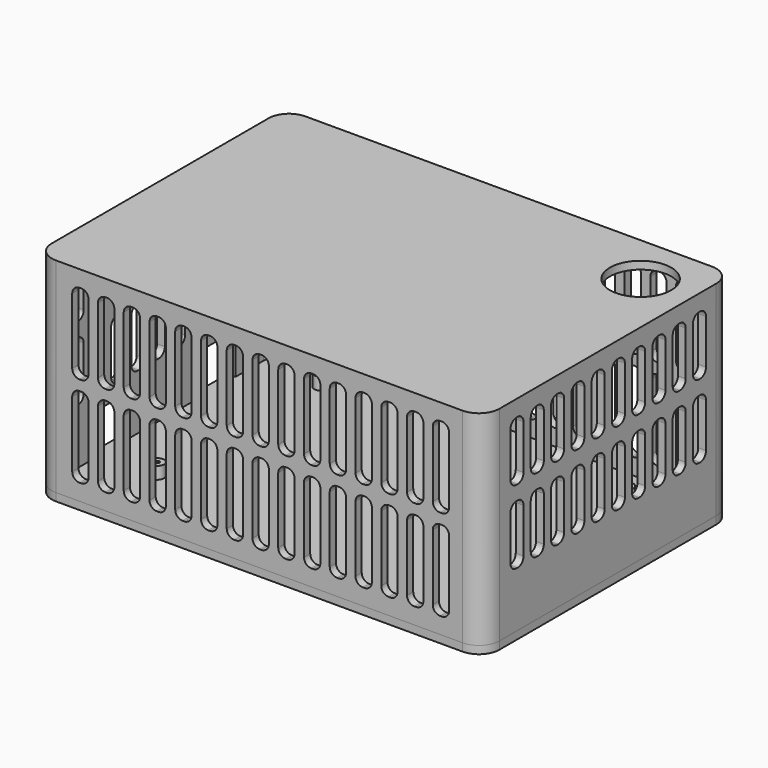
from build123d import *

# Parameters (mm, degrees)
F2_W         = 109.505
F2_H         = 76.3
F3_DEPTH     = 50
F4_T         = -1.905
F5_DEPTH     = 1.905
F0_W         = 9.525
F0_H         = 11.43
F0_W_2       = 6.35
F6_DEPTH     = 10
F0_W_3       = 11.43
F0_H_2       = 8.4328
F0_W_4       = 1.905
F7_DEPTH     = 10
F0_R         = 1.5875
F0_R_2       = 1.59
F8_DEPTH     = 3
F10_D        = 3.3
F12_D        = 1
F12_DEPTH    = 3
F12_TIP      = 0.3004303095
F13_DEPTH    = 5
F14_D        = 1
F14_DEPTH    = 3
F14_TIP      = 0.3004303095
F15_T1_DEPTH = 5
F16_R        = 5
F16_2_R      = 5
F18_DEPTH    = 76.301
F20_DEPTH    = 109.506
F21_R        = 7.5
F22_DEPTH    = 51.906


# Not quite as in the source:
# - a fillet or chamfer that OpenCascade refuses, or shapes differently, is made with other operations: its cross-section is extruded or revolved along the edge and cut away or added


with BuildPart() as f3:
    # F2 (on Top) → F3 (new body)
    with BuildSketch(Plane.XY):
        with Locations((16.3090971484, -6.4307405627)):
            Rectangle(F2_W, F2_H)
    extrude(amount=F3_DEPTH)

    # F4
    f4_openings = [f3.faces().sort_by_distance(p)[0] for p in [
        (16.309097, -6.430741, 0),
    ]]
    offset(amount=F4_T, openings=f4_openings)

    # F0 (on Top) → F6 (cut)
    with BuildSketch(Plane.XY):
        with Locations((-31.7759028516, 8.4792594373)):
            Rectangle(F0_W, F0_H)
        with Locations((-39.7134028516, 8.4792594373)):
            Rectangle(F0_W_2, F0_H)
    extrude(amount=F6_DEPTH, mode=Mode.SUBTRACT)

    # F0 (on Top) → F7 (cut)
    with BuildSketch(Plane.XY):
        with Locations((-30.8234028516, -22.2293405627)):
            Rectangle(F0_W_3, F0_H_2)
        with Locations((-37.4909028516, -22.2293405627)):
            Rectangle(F0_W_4, F0_H_2)
    extrude(amount=F7_DEPTH, mode=Mode.SUBTRACT)

    # F9 (on face) → F13 (join)
    with BuildSketch(Plane.XY):
        with BuildLine():
            ThreePointArc((69.5615971484, 27.7192594373), (67.0615971484, 30.2192594373), (64.5615971484, 27.7192594373))
            Line((64.5615971484, 27.7192594373), (67.0615971484, 27.7192594373))
            Line((67.0615971484, 27.7192594373), (67.0615971484, 25.2192594373))
            ThreePointArc((67.0615971484, 25.2192594373), (68.8293641014, 25.9514924844), (69.5615971484, 27.7192594373))
        make_face()
        with BuildLine():
            Line((67.0615971484, 27.7192594373), (64.5615971484, 27.7192594373))
            ThreePointArc((64.5615971484, 27.7192594373), (65.2938301955, 25.9514924844), (67.0615971484, 25.2192594373))
            Line((67.0615971484, 25.2192594373), (67.0615971484, 27.7192594373))
        make_face()
        with BuildLine():
            Line((67.0615971484, -40.5807405627), (67.0615971484, -38.0807405627))
            ThreePointArc((67.0615971484, -38.0807405627), (65.2938301955, -38.8129736097), (64.5615971484, -40.5807405627))
            Line((64.5615971484, -40.5807405627), (67.0615971484, -40.5807405627))
        make_face()
        with BuildLine():
            ThreePointArc((69.5615971484, -40.5807405627), (68.8293641014, -38.8129736097), (67.0615971484, -38.0807405627))
            Line((67.0615971484, -38.0807405627), (67.0615971484, -40.5807405627))
            Line((67.0615971484, -40.5807405627), (64.5615971484, -40.5807405627))
            ThreePointArc((64.5615971484, -40.5807405627), (67.0615971484, -43.0807405627), (69.5615971484, -40.5807405627))
        make_face()
        with BuildLine():
            Line((-34.4434028516, 27.7192594373), (-31.9434028516, 27.7192594373))
            ThreePointArc((-31.9434028516, 27.7192594373), (-36.2111698045, 29.4870263903), (-34.4434028516, 25.2192594373))
            Line((-34.4434028516, 25.2192594373), (-34.4434028516, 27.7192594373))
        make_face()
        with BuildLine():
            ThreePointArc((-34.4434028516, 25.2192594373), (-32.6756358986, 25.9514924844), (-31.9434028516, 27.7192594373))
            Line((-31.9434028516, 27.7192594373), (-34.4434028516, 27.7192594373))
            Line((-34.4434028516, 27.7192594373), (-34.4434028516, 25.2192594373))
        make_face()
        with BuildLine():
            ThreePointArc((-31.9434028516, -40.5807405627), (-32.6756358986, -38.8129736097), (-34.4434028516, -38.0807405627))
            Line((-34.4434028516, -38.0807405627), (-34.4434028516, -40.5807405627))
            Line((-34.4434028516, -40.5807405627), (-31.9434028516, -40.5807405627))
        make_face()
        with BuildLine():
            Line((-34.4434028516, -40.5807405627), (-34.4434028516, -38.0807405627))
            ThreePointArc((-34.4434028516, -38.0807405627), (-36.2111698045, -42.3485075156), (-31.9434028516, -40.5807405627))
            Line((-31.9434028516, -40.5807405627), (-34.4434028516, -40.5807405627))
        make_face()
    extrude(amount=F13_DEPTH)

    # F14
    with Locations(Plane(origin=(0, 0, 0), x_dir=(1, 0, 0), z_dir=(0, 0, -1))):
        with Locations((-34.4434028516, 40.5807405627), (67.0615971484, 40.5807405627), (-34.4434028516, -27.7192594373), (67.0615971484, -27.7192594373)):
            Hole(F14_D / 2, depth=F14_DEPTH)
            with Locations((0, 0, -(F14_DEPTH + F14_TIP / 2))):  # 118° drill point
                Cone(0, F14_D / 2, F14_TIP, mode=Mode.SUBTRACT)

    # F15: fillet of radius 2.5 on 8 edges, made by hand

    # F15_s2 → F15_t1 (join)
    with BuildSketch(Plane.XY):
        with BuildLine():
            ThreePointArc((66.8590971484, -38.0889553091), (68.494564776, -37.2918307885), (69.1565971484, -35.5971700555))
            Line((69.1565971484, -35.5971700555), (69.1565971484, -39.2165649875))
            ThreePointArc((69.1565971484, -39.2165649875), (68.163080221, -38.3364734126), (66.8590971484, -38.0889553091))
        make_face()
        with BuildLine():
            ThreePointArc((62.0780266412, -42.6757405627), (63.7726873742, -42.0137081902), (64.5698118948, -40.3782405627))
            ThreePointArc((64.5698118948, -40.3782405627), (64.8173299984, -41.6822236353), (65.6974215732, -42.6757405627))
            Line((65.6974215732, -42.6757405627), (62.0780266412, -42.6757405627))
        make_face()
        with BuildLine():
            ThreePointArc((69.1565971484, 22.7356889301), (68.494564776, 24.4303496632), (66.8590971484, 25.2274741837))
            ThreePointArc((66.8590971484, 25.2274741837), (68.163080221, 25.4749922873), (69.1565971484, 26.3550838621))
            Line((69.1565971484, 26.3550838621), (69.1565971484, 22.7356889301))
        make_face()
        with BuildLine():
            ThreePointArc((64.5698118948, 27.5167594373), (63.7726873742, 29.1522270649), (62.0780266412, 29.8142594373))
            Line((62.0780266412, 29.8142594373), (65.6974215732, 29.8142594373))
            ThreePointArc((65.6974215732, 29.8142594373), (64.8173299984, 28.8207425099), (64.5698118948, 27.5167594373))
        make_face()
        with BuildLine():
            ThreePointArc((-36.5384028516, 22.7356889301), (-35.8763704792, 24.4303496632), (-34.2409028516, 25.2274741837))
            ThreePointArc((-34.2409028516, 25.2274741837), (-35.5448859242, 25.4749922873), (-36.5384028516, 26.3550838621))
            Line((-36.5384028516, 26.3550838621), (-36.5384028516, 22.7356889301))
        make_face()
        with BuildLine():
            ThreePointArc((-36.5384028516, -35.5971700555), (-35.8763704792, -37.2918307885), (-34.2409028516, -38.0889553091))
            ThreePointArc((-34.2409028516, -38.0889553091), (-35.5448859242, -38.3364734126), (-36.5384028516, -39.2165649875))
            Line((-36.5384028516, -39.2165649875), (-36.5384028516, -35.5971700555))
        make_face()
        with BuildLine():
            ThreePointArc((-31.951617598, -40.3782405627), (-31.1544930774, -42.0137081902), (-29.4598323444, -42.6757405627))
            Line((-29.4598323444, -42.6757405627), (-33.0792272764, -42.6757405627))
            ThreePointArc((-33.0792272764, -42.6757405627), (-32.1991357015, -41.6822236353), (-31.951617598, -40.3782405627))
        make_face()
        with BuildLine():
            ThreePointArc((-29.4598323444, 29.8142594373), (-31.1544930774, 29.1522270649), (-31.951617598, 27.5167594373))
            ThreePointArc((-31.951617598, 27.5167594373), (-32.1991357015, 28.8207425099), (-33.0792272764, 29.8142594373))
            Line((-33.0792272764, 29.8142594373), (-29.4598323444, 29.8142594373))
        make_face()
    extrude(amount=F15_T1_DEPTH)

    # F16
    f16_edges = [f3.edges().sort_by_distance(p)[0] for p in [
        (-38.443403, -44.580741, 25),
        (71.061597, -44.580741, 25),
        (-38.443403, 31.719259, 25),
        (71.061597, 31.719259, 25),
    ]]
    fillet(f16_edges, radius=F16_R)

    # F17 (on face) → F18 (cut, through all)
    with BuildSketch(Plane.XZ.offset(44.5807405627)):
        with BuildLine():
            Line((-27.2434028516, 46), (-27.6434028516, 46))
            ThreePointArc((-27.6434028516, 46), (-28.9161950577, 45.4727922061), (-29.4434028516, 44.2))
            Line((-29.4434028516, 44.2), (-29.4434028516, 28.05))
            ThreePointArc((-29.4434028516, 28.05), (-28.9161950577, 26.7772077939), (-27.6434028516, 26.25))
            Line((-27.6434028516, 26.25), (-27.2434028516, 26.25))
            ThreePointArc((-27.2434028516, 26.25), (-25.9706106454, 26.7772077939), (-25.4434028516, 28.05))
            Line((-25.4434028516, 28.05), (-25.4434028516, 44.2))
            ThreePointArc((-25.4434028516, 44.2), (-25.9706106454, 45.4727922061), (-27.2434028516, 46))
        make_face()
        with BuildLine():
            Line((-20.9434028516, 46), (-21.3434028516, 46))
            ThreePointArc((-21.3434028516, 46), (-22.6161950577, 45.4727922061), (-23.1434028516, 44.2))
            Line((-23.1434028516, 44.2), (-23.1434028516, 28.05))
            ThreePointArc((-23.1434028516, 28.05), (-22.6161950577, 26.7772077939), (-21.3434028516, 26.25))
            Line((-21.3434028516, 26.25), (-20.9434028516, 26.25))
            ThreePointArc((-20.9434028516, 26.25), (-19.6706106454, 26.7772077939), (-19.1434028516, 28.05))
            Line((-19.1434028516, 28.05), (-19.1434028516, 44.2))
            ThreePointArc((-19.1434028516, 44.2), (-19.6706106454, 45.4727922061), (-20.9434028516, 46))
        make_face()
        with BuildLine():
            Line((-14.6434028516, 46), (-15.0434028516, 46))
            ThreePointArc((-15.0434028516, 46), (-16.3161950577, 45.4727922061), (-16.8434028516, 44.2))
            Line((-16.8434028516, 44.2), (-16.8434028516, 28.05))
            ThreePointArc((-16.8434028516, 28.05), (-16.3161950577, 26.7772077939), (-15.0434028516, 26.25))
            Line((-15.0434028516, 26.25), (-14.6434028516, 26.25))
            ThreePointArc((-14.6434028516, 26.25), (-13.3706106454, 26.7772077939), (-12.8434028516, 28.05))
            Line((-12.8434028516, 28.05), (-12.8434028516, 44.2))
            ThreePointArc((-12.8434028516, 44.2), (-13.3706106454, 45.4727922061), (-14.6434028516, 46))
        make_face()
        with BuildLine():
            Line((-8.3434028516, 46), (-8.7434028516, 46))
            ThreePointArc((-8.7434028516, 46), (-10.0161950577, 45.4727922061), (-10.5434028516, 44.2))
            Line((-10.5434028516, 44.2), (-10.5434028516, 28.05))
            ThreePointArc((-10.5434028516, 28.05), (-10.0161950577, 26.7772077939), (-8.7434028516, 26.25))
            Line((-8.7434028516, 26.25), (-8.3434028516, 26.25))
            ThreePointArc((-8.3434028516, 26.25), (-7.0706106454, 26.7772077939), (-6.5434028516, 28.05))
            Line((-6.5434028516, 28.05), (-6.5434028516, 44.2))
            ThreePointArc((-6.5434028516, 44.2), (-7.0706106454, 45.4727922061), (-8.3434028516, 46))
        make_face()
        with BuildLine():
            Line((-2.0434028516, 46), (-2.4434028516, 46))
            ThreePointArc((-2.4434028516, 46), (-3.7161950577, 45.4727922061), (-4.2434028516, 44.2))
            Line((-4.2434028516, 44.2), (-4.2434028516, 28.05))
            ThreePointArc((-4.2434028516, 28.05), (-3.7161950577, 26.7772077939), (-2.4434028516, 26.25))
            Line((-2.4434028516, 26.25), (-2.0434028516, 26.25))
            ThreePointArc((-2.0434028516, 26.25), (-0.7706106454, 26.7772077939), (-0.2434028516, 28.05))
            Line((-0.2434028516, 28.05), (-0.2434028516, 44.2))
            ThreePointArc((-0.2434028516, 44.2), (-0.7706106454, 45.4727922061), (-2.0434028516, 46))
        make_face()
        with BuildLine():
            Line((4.2565971484, 46), (3.8565971484, 46))
            ThreePointArc((3.8565971484, 46), (2.5838049423, 45.4727922061), (2.0565971484, 44.2))
            Line((2.0565971484, 44.2), (2.0565971484, 28.05))
            ThreePointArc((2.0565971484, 28.05), (2.5838049423, 26.7772077939), (3.8565971484, 26.25))
            Line((3.8565971484, 26.25), (4.2565971484, 26.25))
            ThreePointArc((4.2565971484, 26.25), (5.5293893546, 26.7772077939), (6.0565971484, 28.05))
            Line((6.0565971484, 28.05), (6.0565971484, 44.2))
            ThreePointArc((6.0565971484, 44.2), (5.5293893546, 45.4727922061), (4.2565971484, 46))
        make_face()
        with BuildLine():
            Line((10.5565971484, 46), (10.1565971484, 46))
            ThreePointArc((10.1565971484, 46), (8.8838049423, 45.4727922061), (8.3565971484, 44.2))
            Line((8.3565971484, 44.2), (8.3565971484, 28.05))
            ThreePointArc((8.3565971484, 28.05), (8.8838049423, 26.7772077939), (10.1565971484, 26.25))
            Line((10.1565971484, 26.25), (10.5565971484, 26.25))
            ThreePointArc((10.5565971484, 26.25), (11.8293893546, 26.7772077939), (12.3565971484, 28.05))
            Line((12.3565971484, 28.05), (12.3565971484, 44.2))
            ThreePointArc((12.3565971484, 44.2), (11.8293893546, 45.4727922061), (10.5565971484, 46))
        make_face()
        with BuildLine():
            Line((16.8565971484, 46), (16.4565971484, 46))
            ThreePointArc((16.4565971484, 46), (15.1838049423, 45.4727922061), (14.6565971484, 44.2))
            Line((14.6565971484, 44.2), (14.6565971484, 28.05))
            ThreePointArc((14.6565971484, 28.05), (15.1838049423, 26.7772077939), (16.4565971484, 26.25))
            Line((16.4565971484, 26.25), (16.8565971484, 26.25))
            ThreePointArc((16.8565971484, 26.25), (18.1293893546, 26.7772077939), (18.6565971484, 28.05))
            Line((18.6565971484, 28.05), (18.6565971484, 44.2))
            ThreePointArc((18.6565971484, 44.2), (18.1293893546, 45.4727922061), (16.8565971484, 46))
        make_face()
        with BuildLine():
            Line((23.1565971484, 46), (22.7565971484, 46))
            ThreePointArc((22.7565971484, 46), (21.4838049423, 45.4727922061), (20.9565971484, 44.2))
            Line((20.9565971484, 44.2), (20.9565971484, 28.05))
            ThreePointArc((20.9565971484, 28.05), (21.4838049423, 26.7772077939), (22.7565971484, 26.25))
            Line((22.7565971484, 26.25), (23.1565971484, 26.25))
            ThreePointArc((23.1565971484, 26.25), (24.4293893546, 26.7772077939), (24.9565971484, 28.05))
            Line((24.9565971484, 28.05), (24.9565971484, 44.2))
            ThreePointArc((24.9565971484, 44.2), (24.4293893546, 45.4727922061), (23.1565971484, 46))
        make_face()
        with BuildLine():
            Line((29.4565971484, 46), (29.0565971484, 46))
            ThreePointArc((29.0565971484, 46), (27.7838049423, 45.4727922061), (27.2565971484, 44.2))
            Line((27.2565971484, 44.2), (27.2565971484, 28.05))
            ThreePointArc((27.2565971484, 28.05), (27.7838049423, 26.7772077939), (29.0565971484, 26.25))
            Line((29.0565971484, 26.25), (29.4565971484, 26.25))
            ThreePointArc((29.4565971484, 26.25), (30.7293893546, 26.7772077939), (31.2565971484, 28.05))
            Line((31.2565971484, 28.05), (31.2565971484, 44.2))
            ThreePointArc((31.2565971484, 44.2), (30.7293893546, 45.4727922061), (29.4565971484, 46))
        make_face()
        with BuildLine():
            Line((35.7565971484, 46), (35.3565971484, 46))
            ThreePointArc((35.3565971484, 46), (34.0838049423, 45.4727922061), (33.5565971484, 44.2))
            Line((33.5565971484, 44.2), (33.5565971484, 28.05))
            ThreePointArc((33.5565971484, 28.05), (34.0838049423, 26.7772077939), (35.3565971484, 26.25))
            Line((35.3565971484, 26.25), (35.7565971484, 26.25))
            ThreePointArc((35.7565971484, 26.25), (37.0293893546, 26.7772077939), (37.5565971484, 28.05))
            Line((37.5565971484, 28.05), (37.5565971484, 44.2))
            ThreePointArc((37.5565971484, 44.2), (37.0293893546, 45.4727922061), (35.7565971484, 46))
        make_face()
        with BuildLine():
            Line((42.0565971484, 46), (41.6565971484, 46))
            ThreePointArc((41.6565971484, 46), (40.3838049423, 45.4727922061), (39.8565971484, 44.2))
            Line((39.8565971484, 44.2), (39.8565971484, 28.05))
            ThreePointArc((39.8565971484, 28.05), (40.3838049423, 26.7772077939), (41.6565971484, 26.25))
            Line((41.6565971484, 26.25), (42.0565971484, 26.25))
            ThreePointArc((42.0565971484, 26.25), (43.3293893546, 26.7772077939), (43.8565971484, 28.05))
            Line((43.8565971484, 28.05), (43.8565971484, 44.2))
            ThreePointArc((43.8565971484, 44.2), (43.3293893546, 45.4727922061), (42.0565971484, 46))
        make_face()
        with BuildLine():
            Line((48.3565971484, 46), (47.9565971484, 46))
            ThreePointArc((47.9565971484, 46), (46.6838049423, 45.4727922061), (46.1565971484, 44.2))
            Line((46.1565971484, 44.2), (46.1565971484, 28.05))
            ThreePointArc((46.1565971484, 28.05), (46.6838049423, 26.7772077939), (47.9565971484, 26.25))
            Line((47.9565971484, 26.25), (48.3565971484, 26.25))
            ThreePointArc((48.3565971484, 26.25), (49.6293893546, 26.7772077939), (50.1565971484, 28.05))
            Line((50.1565971484, 28.05), (50.1565971484, 44.2))
            ThreePointArc((50.1565971484, 44.2), (49.6293893546, 45.4727922061), (48.3565971484, 46))
        make_face()
        with BuildLine():
            Line((54.6565971484, 46), (54.2565971484, 46))
            ThreePointArc((54.2565971484, 46), (52.9838049423, 45.4727922061), (52.4565971484, 44.2))
            Line((52.4565971484, 44.2), (52.4565971484, 28.05))
            ThreePointArc((52.4565971484, 28.05), (52.9838049423, 26.7772077939), (54.2565971484, 26.25))
            Line((54.2565971484, 26.25), (54.6565971484, 26.25))
            ThreePointArc((54.6565971484, 26.25), (55.9293893546, 26.7772077939), (56.4565971484, 28.05))
            Line((56.4565971484, 28.05), (56.4565971484, 44.2))
            ThreePointArc((56.4565971484, 44.2), (55.9293893546, 45.4727922061), (54.6565971484, 46))
        make_face()
        with BuildLine():
            Line((60.9565971484, 46), (60.5565971484, 46))
            ThreePointArc((60.5565971484, 46), (59.2838049423, 45.4727922061), (58.7565971484, 44.2))
            Line((58.7565971484, 44.2), (58.7565971484, 28.05))
            ThreePointArc((58.7565971484, 28.05), (59.2838049423, 26.7772077939), (60.5565971484, 26.25))
            Line((60.5565971484, 26.25), (60.9565971484, 26.25))
            ThreePointArc((60.9565971484, 26.25), (62.2293893546, 26.7772077939), (62.7565971484, 28.05))
            Line((62.7565971484, 28.05), (62.7565971484, 44.2))
            ThreePointArc((62.7565971484, 44.2), (62.2293893546, 45.4727922061), (60.9565971484, 46))
        make_face()
        with BuildLine():
            Line((-27.2434028516, 23.75), (-27.6434028516, 23.75))
            ThreePointArc((-27.6434028516, 23.75), (-28.9161950577, 23.2227922061), (-29.4434028516, 21.95))
            Line((-29.4434028516, 21.95), (-29.4434028516, 5.8))
            ThreePointArc((-29.4434028516, 5.8), (-28.9161950577, 4.5272077939), (-27.6434028516, 4))
            Line((-27.6434028516, 4), (-27.2434028516, 4))
            ThreePointArc((-27.2434028516, 4), (-25.9706106454, 4.5272077939), (-25.4434028516, 5.8))
            Line((-25.4434028516, 5.8), (-25.4434028516, 21.95))
            ThreePointArc((-25.4434028516, 21.95), (-25.9706106454, 23.2227922061), (-27.2434028516, 23.75))
        make_face()
        with BuildLine():
            Line((-20.9434028516, 23.75), (-21.3434028516, 23.75))
            ThreePointArc((-21.3434028516, 23.75), (-22.6161950577, 23.2227922061), (-23.1434028516, 21.95))
            Line((-23.1434028516, 21.95), (-23.1434028516, 5.8))
            ThreePointArc((-23.1434028516, 5.8), (-22.6161950577, 4.5272077939), (-21.3434028516, 4))
            Line((-21.3434028516, 4), (-20.9434028516, 4))
            ThreePointArc((-20.9434028516, 4), (-19.6706106454, 4.5272077939), (-19.1434028516, 5.8))
            Line((-19.1434028516, 5.8), (-19.1434028516, 21.95))
            ThreePointArc((-19.1434028516, 21.95), (-19.6706106454, 23.2227922061), (-20.9434028516, 23.75))
        make_face()
        with BuildLine():
            Line((-14.6434028516, 23.75), (-15.0434028516, 23.75))
            ThreePointArc((-15.0434028516, 23.75), (-16.3161950577, 23.2227922061), (-16.8434028516, 21.95))
            Line((-16.8434028516, 21.95), (-16.8434028516, 5.8))
            ThreePointArc((-16.8434028516, 5.8), (-16.3161950577, 4.5272077939), (-15.0434028516, 4))
            Line((-15.0434028516, 4), (-14.6434028516, 4))
            ThreePointArc((-14.6434028516, 4), (-13.3706106454, 4.5272077939), (-12.8434028516, 5.8))
            Line((-12.8434028516, 5.8), (-12.8434028516, 21.95))
            ThreePointArc((-12.8434028516, 21.95), (-13.3706106454, 23.2227922061), (-14.6434028516, 23.75))
        make_face()
        with BuildLine():
            Line((-8.3434028516, 23.75), (-8.7434028516, 23.75))
            ThreePointArc((-8.7434028516, 23.75), (-10.0161950577, 23.2227922061), (-10.5434028516, 21.95))
            Line((-10.5434028516, 21.95), (-10.5434028516, 5.8))
            ThreePointArc((-10.5434028516, 5.8), (-10.0161950577, 4.5272077939), (-8.7434028516, 4))
            Line((-8.7434028516, 4), (-8.3434028516, 4))
            ThreePointArc((-8.3434028516, 4), (-7.0706106454, 4.5272077939), (-6.5434028516, 5.8))
            Line((-6.5434028516, 5.8), (-6.5434028516, 21.95))
            ThreePointArc((-6.5434028516, 21.95), (-7.0706106454, 23.2227922061), (-8.3434028516, 23.75))
        make_face()
        with BuildLine():
            Line((-2.0434028516, 23.75), (-2.4434028516, 23.75))
            ThreePointArc((-2.4434028516, 23.75), (-3.7161950577, 23.2227922061), (-4.2434028516, 21.95))
            Line((-4.2434028516, 21.95), (-4.2434028516, 5.8))
            ThreePointArc((-4.2434028516, 5.8), (-3.7161950577, 4.5272077939), (-2.4434028516, 4))
            Line((-2.4434028516, 4), (-2.0434028516, 4))
            ThreePointArc((-2.0434028516, 4), (-0.7706106454, 4.5272077939), (-0.2434028516, 5.8))
            Line((-0.2434028516, 5.8), (-0.2434028516, 21.95))
            ThreePointArc((-0.2434028516, 21.95), (-0.7706106454, 23.2227922061), (-2.0434028516, 23.75))
        make_face()
        with BuildLine():
            Line((4.2565971484, 23.75), (3.8565971484, 23.75))
            ThreePointArc((3.8565971484, 23.75), (2.5838049423, 23.2227922061), (2.0565971484, 21.95))
            Line((2.0565971484, 21.95), (2.0565971484, 5.8))
            ThreePointArc((2.0565971484, 5.8), (2.5838049423, 4.5272077939), (3.8565971484, 4))
            Line((3.8565971484, 4), (4.2565971484, 4))
            ThreePointArc((4.2565971484, 4), (5.5293893546, 4.5272077939), (6.0565971484, 5.8))
            Line((6.0565971484, 5.8), (6.0565971484, 21.95))
            ThreePointArc((6.0565971484, 21.95), (5.5293893546, 23.2227922061), (4.2565971484, 23.75))
        make_face()
        with BuildLine():
            Line((10.5565971484, 23.75), (10.1565971484, 23.75))
            ThreePointArc((10.1565971484, 23.75), (8.8838049423, 23.2227922061), (8.3565971484, 21.95))
            Line((8.3565971484, 21.95), (8.3565971484, 5.8))
            ThreePointArc((8.3565971484, 5.8), (8.8838049423, 4.5272077939), (10.1565971484, 4))
            Line((10.1565971484, 4), (10.5565971484, 4))
            ThreePointArc((10.5565971484, 4), (11.8293893546, 4.5272077939), (12.3565971484, 5.8))
            Line((12.3565971484, 5.8), (12.3565971484, 21.95))
            ThreePointArc((12.3565971484, 21.95), (11.8293893546, 23.2227922061), (10.5565971484, 23.75))
        make_face()
        with BuildLine():
            Line((16.8565971484, 23.75), (16.4565971484, 23.75))
            ThreePointArc((16.4565971484, 23.75), (15.1838049423, 23.2227922061), (14.6565971484, 21.95))
            Line((14.6565971484, 21.95), (14.6565971484, 5.8))
            ThreePointArc((14.6565971484, 5.8), (15.1838049423, 4.5272077939), (16.4565971484, 4))
            Line((16.4565971484, 4), (16.8565971484, 4))
            ThreePointArc((16.8565971484, 4), (18.1293893546, 4.5272077939), (18.6565971484, 5.8))
            Line((18.6565971484, 5.8), (18.6565971484, 21.95))
            ThreePointArc((18.6565971484, 21.95), (18.1293893546, 23.2227922061), (16.8565971484, 23.75))
        make_face()
        with BuildLine():
            Line((23.1565971484, 23.75), (22.7565971484, 23.75))
            ThreePointArc((22.7565971484, 23.75), (21.4838049423, 23.2227922061), (20.9565971484, 21.95))
            Line((20.9565971484, 21.95), (20.9565971484, 5.8))
            ThreePointArc((20.9565971484, 5.8), (21.4838049423, 4.5272077939), (22.7565971484, 4))
            Line((22.7565971484, 4), (23.1565971484, 4))
            ThreePointArc((23.1565971484, 4), (24.4293893546, 4.5272077939), (24.9565971484, 5.8))
            Line((24.9565971484, 5.8), (24.9565971484, 21.95))
            ThreePointArc((24.9565971484, 21.95), (24.4293893546, 23.2227922061), (23.1565971484, 23.75))
        make_face()
        with BuildLine():
            Line((29.4565971484, 23.75), (29.0565971484, 23.75))
            ThreePointArc((29.0565971484, 23.75), (27.7838049423, 23.2227922061), (27.2565971484, 21.95))
            Line((27.2565971484, 21.95), (27.2565971484, 5.8))
            ThreePointArc((27.2565971484, 5.8), (27.7838049423, 4.5272077939), (29.0565971484, 4))
            Line((29.0565971484, 4), (29.4565971484, 4))
            ThreePointArc((29.4565971484, 4), (30.7293893546, 4.5272077939), (31.2565971484, 5.8))
            Line((31.2565971484, 5.8), (31.2565971484, 21.95))
            ThreePointArc((31.2565971484, 21.95), (30.7293893546, 23.2227922061), (29.4565971484, 23.75))
        make_face()
        with BuildLine():
            Line((35.7565971484, 23.75), (35.3565971484, 23.75))
            ThreePointArc((35.3565971484, 23.75), (34.0838049423, 23.2227922061), (33.5565971484, 21.95))
            Line((33.5565971484, 21.95), (33.5565971484, 5.8))
            ThreePointArc((33.5565971484, 5.8), (34.0838049423, 4.5272077939), (35.3565971484, 4))
            Line((35.3565971484, 4), (35.7565971484, 4))
            ThreePointArc((35.7565971484, 4), (37.0293893546, 4.5272077939), (37.5565971484, 5.8))
            Line((37.5565971484, 5.8), (37.5565971484, 21.95))
            ThreePointArc((37.5565971484, 21.95), (37.0293893546, 23.2227922061), (35.7565971484, 23.75))
        make_face()
        with BuildLine():
            Line((42.0565971484, 23.75), (41.6565971484, 23.75))
            ThreePointArc((41.6565971484, 23.75), (40.3838049423, 23.2227922061), (39.8565971484, 21.95))
            Line((39.8565971484, 21.95), (39.8565971484, 5.8))
            ThreePointArc((39.8565971484, 5.8), (40.3838049423, 4.5272077939), (41.6565971484, 4))
            Line((41.6565971484, 4), (42.0565971484, 4))
            ThreePointArc((42.0565971484, 4), (43.3293893546, 4.5272077939), (43.8565971484, 5.8))
            Line((43.8565971484, 5.8), (43.8565971484, 21.95))
            ThreePointArc((43.8565971484, 21.95), (43.3293893546, 23.2227922061), (42.0565971484, 23.75))
        make_face()
        with BuildLine():
            Line((48.3565971484, 23.75), (47.9565971484, 23.75))
            ThreePointArc((47.9565971484, 23.75), (46.6838049423, 23.2227922061), (46.1565971484, 21.95))
            Line((46.1565971484, 21.95), (46.1565971484, 5.8))
            ThreePointArc((46.1565971484, 5.8), (46.6838049423, 4.5272077939), (47.9565971484, 4))
            Line((47.9565971484, 4), (48.3565971484, 4))
            ThreePointArc((48.3565971484, 4), (49.6293893546, 4.5272077939), (50.1565971484, 5.8))
            Line((50.1565971484, 5.8), (50.1565971484, 21.95))
            ThreePointArc((50.1565971484, 21.95), (49.6293893546, 23.2227922061), (48.3565971484, 23.75))
        make_face()
        with BuildLine():
            Line((54.6565971484, 23.75), (54.2565971484, 23.75))
            ThreePointArc((54.2565971484, 23.75), (52.9838049423, 23.2227922061), (52.4565971484, 21.95))
            Line((52.4565971484, 21.95), (52.4565971484, 5.8))
            ThreePointArc((52.4565971484, 5.8), (52.9838049423, 4.5272077939), (54.2565971484, 4))
            Line((54.2565971484, 4), (54.6565971484, 4))
            ThreePointArc((54.6565971484, 4), (55.9293893546, 4.5272077939), (56.4565971484, 5.8))
            Line((56.4565971484, 5.8), (56.4565971484, 21.95))
            ThreePointArc((56.4565971484, 21.95), (55.9293893546, 23.2227922061), (54.6565971484, 23.75))
        make_face()
        with BuildLine():
            Line((60.9565971484, 23.75), (60.5565971484, 23.75))
            ThreePointArc((60.5565971484, 23.75), (59.2838049423, 23.2227922061), (58.7565971484, 21.95))
            Line((58.7565971484, 21.95), (58.7565971484, 5.8))
            ThreePointArc((58.7565971484, 5.8), (59.2838049423, 4.5272077939), (60.5565971484, 4))
            Line((60.5565971484, 4), (60.9565971484, 4))
            ThreePointArc((60.9565971484, 4), (62.2293893546, 4.5272077939), (62.7565971484, 5.8))
            Line((62.7565971484, 5.8), (62.7565971484, 21.95))
            ThreePointArc((62.7565971484, 21.95), (62.2293893546, 23.2227922061), (60.9565971484, 23.75))
        make_face()
    extrude(amount=-F18_DEPTH, mode=Mode.SUBTRACT)

    # F19 (on face) → F20 (cut, through all)
    with BuildSketch(Plane(origin=(-38.4434028516, 0, 0), x_dir=(0, -1, 0), z_dir=(-1, 0, 0))):
        with BuildLine():
            Line((-21.400732252, 46), (-21.800732252, 46))
            ThreePointArc((-21.800732252, 46), (-23.0735244581, 45.4727922061), (-23.600732252, 44.2))
            Line((-23.600732252, 44.2), (-23.600732252, 33.3))
            ThreePointArc((-23.600732252, 33.3), (-23.0735244581, 32.0272077939), (-21.800732252, 31.5))
            Line((-21.800732252, 31.5), (-21.400732252, 31.5))
            ThreePointArc((-21.400732252, 31.5), (-20.1279400459, 32.0272077939), (-19.600732252, 33.3))
            Line((-19.600732252, 33.3), (-19.600732252, 44.2))
            ThreePointArc((-19.600732252, 44.2), (-20.1279400459, 45.4727922061), (-21.400732252, 46))
        make_face()
        with BuildLine():
            Line((-13.400732252, 33.3), (-13.400732252, 44.2))
            ThreePointArc((-13.400732252, 44.2), (-13.9279400459, 45.4727922061), (-15.200732252, 46))
            Line((-15.200732252, 46), (-15.600732252, 46))
            ThreePointArc((-15.600732252, 46), (-16.8735244581, 45.4727922061), (-17.400732252, 44.2))
            Line((-17.400732252, 44.2), (-17.400732252, 33.3))
            ThreePointArc((-17.400732252, 33.3), (-16.8735244581, 32.0272077939), (-15.600732252, 31.5))
            Line((-15.600732252, 31.5), (-15.200732252, 31.5))
            ThreePointArc((-15.200732252, 31.5), (-13.9279400459, 32.0272077939), (-13.400732252, 33.3))
        make_face()
        with BuildLine():
            Line((-7.200732252, 33.3), (-7.200732252, 44.2))
            ThreePointArc((-7.200732252, 44.2), (-7.7279400459, 45.4727922061), (-9.000732252, 46))
            Line((-9.000732252, 46), (-9.400732252, 46))
            ThreePointArc((-9.400732252, 46), (-10.6735244581, 45.4727922061), (-11.200732252, 44.2))
            Line((-11.200732252, 44.2), (-11.200732252, 33.3))
            ThreePointArc((-11.200732252, 33.3), (-10.6735244581, 32.0272077939), (-9.400732252, 31.5))
            Line((-9.400732252, 31.5), (-9.000732252, 31.5))
            ThreePointArc((-9.000732252, 31.5), (-7.7279400459, 32.0272077939), (-7.200732252, 33.3))
        make_face()
        with BuildLine():
            Line((-1.000732252, 33.3), (-1.000732252, 44.2))
            ThreePointArc((-1.000732252, 44.2), (-1.5279400459, 45.4727922061), (-2.800732252, 46))
            Line((-2.800732252, 46), (-3.200732252, 46))
            ThreePointArc((-3.200732252, 46), (-4.4735244581, 45.4727922061), (-5.000732252, 44.2))
            Line((-5.000732252, 44.2), (-5.000732252, 33.3))
            ThreePointArc((-5.000732252, 33.3), (-4.4735244581, 32.0272077939), (-3.200732252, 31.5))
            Line((-3.200732252, 31.5), (-2.800732252, 31.5))
            ThreePointArc((-2.800732252, 31.5), (-1.5279400459, 32.0272077939), (-1.000732252, 33.3))
        make_face()
        with BuildLine():
            Line((5.199267748, 33.3), (5.199267748, 44.2))
            ThreePointArc((5.199267748, 44.2), (4.6720599541, 45.4727922061), (3.399267748, 46))
            Line((3.399267748, 46), (2.999267748, 46))
            ThreePointArc((2.999267748, 46), (1.7264755419, 45.4727922061), (1.199267748, 44.2))
            Line((1.199267748, 44.2), (1.199267748, 33.3))
            ThreePointArc((1.199267748, 33.3), (1.7264755419, 32.0272077939), (2.999267748, 31.5))
            Line((2.999267748, 31.5), (3.399267748, 31.5))
            ThreePointArc((3.399267748, 31.5), (4.6720599541, 32.0272077939), (5.199267748, 33.3))
        make_face()
        with BuildLine():
            Line((11.399267748, 33.3), (11.399267748, 44.2))
            ThreePointArc((11.399267748, 44.2), (10.8720599541, 45.4727922061), (9.599267748, 46))
            Line((9.599267748, 46), (9.199267748, 46))
            ThreePointArc((9.199267748, 46), (7.9264755419, 45.4727922061), (7.399267748, 44.2))
            Line((7.399267748, 44.2), (7.399267748, 33.3))
            ThreePointArc((7.399267748, 33.3), (7.9264755419, 32.0272077939), (9.199267748, 31.5))
            Line((9.199267748, 31.5), (9.599267748, 31.5))
            ThreePointArc((9.599267748, 31.5), (10.8720599541, 32.0272077939), (11.399267748, 33.3))
        make_face()
        with BuildLine():
            Line((17.599267748, 33.3), (17.599267748, 44.2))
            ThreePointArc((17.599267748, 44.2), (17.0720599541, 45.4727922061), (15.799267748, 46))
            Line((15.799267748, 46), (15.399267748, 46))
            ThreePointArc((15.399267748, 46), (14.1264755419, 45.4727922061), (13.599267748, 44.2))
            Line((13.599267748, 44.2), (13.599267748, 33.3))
            ThreePointArc((13.599267748, 33.3), (14.1264755419, 32.0272077939), (15.399267748, 31.5))
            Line((15.399267748, 31.5), (15.799267748, 31.5))
            ThreePointArc((15.799267748, 31.5), (17.0720599541, 32.0272077939), (17.599267748, 33.3))
        make_face()
        with BuildLine():
            Line((23.799267748, 33.3), (23.799267748, 44.2))
            ThreePointArc((23.799267748, 44.2), (23.2720599541, 45.4727922061), (21.999267748, 46))
            Line((21.999267748, 46), (21.599267748, 46))
            ThreePointArc((21.599267748, 46), (20.3264755419, 45.4727922061), (19.799267748, 44.2))
            Line((19.799267748, 44.2), (19.799267748, 33.3))
            ThreePointArc((19.799267748, 33.3), (20.3264755419, 32.0272077939), (21.599267748, 31.5))
            Line((21.599267748, 31.5), (21.999267748, 31.5))
            ThreePointArc((21.999267748, 31.5), (23.2720599541, 32.0272077939), (23.799267748, 33.3))
        make_face()
        with BuildLine():
            Line((29.999267748, 33.3), (29.999267748, 44.2))
            ThreePointArc((29.999267748, 44.2), (29.4720599541, 45.4727922061), (28.199267748, 46))
            Line((28.199267748, 46), (27.799267748, 46))
            ThreePointArc((27.799267748, 46), (26.5264755419, 45.4727922061), (25.999267748, 44.2))
            Line((25.999267748, 44.2), (25.999267748, 33.3))
            ThreePointArc((25.999267748, 33.3), (26.5264755419, 32.0272077939), (27.799267748, 31.5))
            Line((27.799267748, 31.5), (28.199267748, 31.5))
            ThreePointArc((28.199267748, 31.5), (29.4720599541, 32.0272077939), (29.999267748, 33.3))
        make_face()
        with BuildLine():
            Line((36.199267748, 33.3), (36.199267748, 44.2))
            ThreePointArc((36.199267748, 44.2), (35.6720599541, 45.4727922061), (34.399267748, 46))
            Line((34.399267748, 46), (33.999267748, 46))
            ThreePointArc((33.999267748, 46), (32.7264755419, 45.4727922061), (32.199267748, 44.2))
            Line((32.199267748, 44.2), (32.199267748, 33.3))
            ThreePointArc((32.199267748, 33.3), (32.7264755419, 32.0272077939), (33.999267748, 31.5))
            Line((33.999267748, 31.5), (34.399267748, 31.5))
            ThreePointArc((34.399267748, 31.5), (35.6720599541, 32.0272077939), (36.199267748, 33.3))
        make_face()
        with BuildLine():
            Line((-19.600732252, 15.3), (-19.600732252, 26.2))
            ThreePointArc((-19.600732252, 26.2), (-20.1279400459, 27.4727922061), (-21.400732252, 28))
            Line((-21.400732252, 28), (-21.800732252, 28))
            ThreePointArc((-21.800732252, 28), (-23.0735244581, 27.4727922061), (-23.600732252, 26.2))
            Line((-23.600732252, 26.2), (-23.600732252, 15.3))
            ThreePointArc((-23.600732252, 15.3), (-23.0735244581, 14.0272077939), (-21.800732252, 13.5))
            Line((-21.800732252, 13.5), (-21.400732252, 13.5))
            ThreePointArc((-21.400732252, 13.5), (-20.1279400459, 14.0272077939), (-19.600732252, 15.3))
        make_face()
        with BuildLine():
            Line((-13.400732252, 15.3), (-13.400732252, 26.2))
            ThreePointArc((-13.400732252, 26.2), (-13.9279400459, 27.4727922061), (-15.200732252, 28))
            Line((-15.200732252, 28), (-15.600732252, 28))
            ThreePointArc((-15.600732252, 28), (-16.8735244581, 27.4727922061), (-17.400732252, 26.2))
            Line((-17.400732252, 26.2), (-17.400732252, 15.3))
            ThreePointArc((-17.400732252, 15.3), (-16.8735244581, 14.0272077939), (-15.600732252, 13.5))
            Line((-15.600732252, 13.5), (-15.200732252, 13.5))
            ThreePointArc((-15.200732252, 13.5), (-13.9279400459, 14.0272077939), (-13.400732252, 15.3))
        make_face()
        with BuildLine():
            Line((-7.200732252, 15.3), (-7.200732252, 26.2))
            ThreePointArc((-7.200732252, 26.2), (-7.7279400459, 27.4727922061), (-9.000732252, 28))
            Line((-9.000732252, 28), (-9.400732252, 28))
            ThreePointArc((-9.400732252, 28), (-10.6735244581, 27.4727922061), (-11.200732252, 26.2))
            Line((-11.200732252, 26.2), (-11.200732252, 15.3))
            ThreePointArc((-11.200732252, 15.3), (-10.6735244581, 14.0272077939), (-9.400732252, 13.5))
            Line((-9.400732252, 13.5), (-9.000732252, 13.5))
            ThreePointArc((-9.000732252, 13.5), (-7.7279400459, 14.0272077939), (-7.200732252, 15.3))
        make_face()
        with BuildLine():
            Line((-1.000732252, 15.3), (-1.000732252, 26.2))
            ThreePointArc((-1.000732252, 26.2), (-1.5279400459, 27.4727922061), (-2.800732252, 28))
            Line((-2.800732252, 28), (-3.200732252, 28))
            ThreePointArc((-3.200732252, 28), (-4.4735244581, 27.4727922061), (-5.000732252, 26.2))
            Line((-5.000732252, 26.2), (-5.000732252, 15.3))
            ThreePointArc((-5.000732252, 15.3), (-4.4735244581, 14.0272077939), (-3.200732252, 13.5))
            Line((-3.200732252, 13.5), (-2.800732252, 13.5))
            ThreePointArc((-2.800732252, 13.5), (-1.5279400459, 14.0272077939), (-1.000732252, 15.3))
        make_face()
        with BuildLine():
            Line((5.199267748, 15.3), (5.199267748, 26.2))
            ThreePointArc((5.199267748, 26.2), (4.6720599541, 27.4727922061), (3.399267748, 28))
            Line((3.399267748, 28), (2.999267748, 28))
            ThreePointArc((2.999267748, 28), (1.7264755419, 27.4727922061), (1.199267748, 26.2))
            Line((1.199267748, 26.2), (1.199267748, 15.3))
            ThreePointArc((1.199267748, 15.3), (1.7264755419, 14.0272077939), (2.999267748, 13.5))
            Line((2.999267748, 13.5), (3.399267748, 13.5))
            ThreePointArc((3.399267748, 13.5), (4.6720599541, 14.0272077939), (5.199267748, 15.3))
        make_face()
        with BuildLine():
            Line((11.399267748, 15.3), (11.399267748, 26.2))
            ThreePointArc((11.399267748, 26.2), (10.8720599541, 27.4727922061), (9.599267748, 28))
            Line((9.599267748, 28), (9.199267748, 28))
            ThreePointArc((9.199267748, 28), (7.9264755419, 27.4727922061), (7.399267748, 26.2))
            Line((7.399267748, 26.2), (7.399267748, 15.3))
            ThreePointArc((7.399267748, 15.3), (7.9264755419, 14.0272077939), (9.199267748, 13.5))
            Line((9.199267748, 13.5), (9.599267748, 13.5))
            ThreePointArc((9.599267748, 13.5), (10.8720599541, 14.0272077939), (11.399267748, 15.3))
        make_face()
        with BuildLine():
            Line((17.599267748, 15.3), (17.599267748, 26.2))
            ThreePointArc((17.599267748, 26.2), (17.0720599541, 27.4727922061), (15.799267748, 28))
            Line((15.799267748, 28), (15.399267748, 28))
            ThreePointArc((15.399267748, 28), (14.1264755419, 27.4727922061), (13.599267748, 26.2))
            Line((13.599267748, 26.2), (13.599267748, 15.3))
            ThreePointArc((13.599267748, 15.3), (14.1264755419, 14.0272077939), (15.399267748, 13.5))
            Line((15.399267748, 13.5), (15.799267748, 13.5))
            ThreePointArc((15.799267748, 13.5), (17.0720599541, 14.0272077939), (17.599267748, 15.3))
        make_face()
        with BuildLine():
            Line((23.799267748, 15.3), (23.799267748, 26.2))
            ThreePointArc((23.799267748, 26.2), (23.2720599541, 27.4727922061), (21.999267748, 28))
            Line((21.999267748, 28), (21.599267748, 28))
            ThreePointArc((21.599267748, 28), (20.3264755419, 27.4727922061), (19.799267748, 26.2))
            Line((19.799267748, 26.2), (19.799267748, 15.3))
            ThreePointArc((19.799267748, 15.3), (20.3264755419, 14.0272077939), (21.599267748, 13.5))
            Line((21.599267748, 13.5), (21.999267748, 13.5))
            ThreePointArc((21.999267748, 13.5), (23.2720599541, 14.0272077939), (23.799267748, 15.3))
        make_face()
        with BuildLine():
            Line((29.999267748, 15.3), (29.999267748, 26.2))
            ThreePointArc((29.999267748, 26.2), (29.4720599541, 27.4727922061), (28.199267748, 28))
            Line((28.199267748, 28), (27.799267748, 28))
            ThreePointArc((27.799267748, 28), (26.5264755419, 27.4727922061), (25.999267748, 26.2))
            Line((25.999267748, 26.2), (25.999267748, 15.3))
            ThreePointArc((25.999267748, 15.3), (26.5264755419, 14.0272077939), (27.799267748, 13.5))
            Line((27.799267748, 13.5), (28.199267748, 13.5))
            ThreePointArc((28.199267748, 13.5), (29.4720599541, 14.0272077939), (29.999267748, 15.3))
        make_face()
        with BuildLine():
            Line((36.199267748, 15.3), (36.199267748, 26.2))
            ThreePointArc((36.199267748, 26.2), (35.6720599541, 27.4727922061), (34.399267748, 28))
            Line((34.399267748, 28), (33.999267748, 28))
            ThreePointArc((33.999267748, 28), (32.7264755419, 27.4727922061), (32.199267748, 26.2))
            Line((32.199267748, 26.2), (32.199267748, 15.3))
            ThreePointArc((32.199267748, 15.3), (32.7264755419, 14.0272077939), (33.999267748, 13.5))
            Line((33.999267748, 13.5), (34.399267748, 13.5))
            ThreePointArc((34.399267748, 13.5), (35.6720599541, 14.0272077939), (36.199267748, 15.3))
        make_face()
    extrude(amount=-F20_DEPTH, mode=Mode.SUBTRACT)

    # F21 (on face) → F22 (cut, through all)
    with BuildSketch(Plane.XY.offset(50)):
        with Locations((58.5615971484, 19.2192594373)):
            Circle(F21_R)
    extrude(amount=-F22_DEPTH, mode=Mode.SUBTRACT)


with BuildPart() as f5:
    # F2 (on Top) → F5 (new body)
    with BuildSketch(Plane.XY):
        with Locations((16.3090971484, -6.4307405627)):
            Rectangle(F2_W, F2_H)
    extrude(amount=-F5_DEPTH)

    # F0 (on Top) → F8 (join)
    with BuildSketch(Plane.XY):
        with Locations((-21.2984028516, 21.1792594373)):
            Circle(F0_R)
        with Locations((-22.5684028516, -27.0807405627)):
            Circle(F0_R_2)
        with Locations((53.6315971484, 21.1792594373)):
            Circle(F0_R_2)
        with Locations((59.9815971484, -27.0807405627)):
            Circle(F0_R_2)
    extrude(amount=F8_DEPTH)

    # F10 (through all)
    with Locations(Plane.XY):
        with Locations((-34.4434028516, 27.7192594373), (67.0615971484, 27.7192594373), (67.0615971484, -40.5807405627), (-34.4434028516, -40.5807405627)):
            Hole(F10_D / 2)

    # F12
    with Locations(Plane.XY.offset(3)):
        with Locations((-22.5684028516, -27.0807405627), (-21.2984028516, 21.1792594373), (59.9815971484, -27.0807405627), (53.6315971484, 21.1792594373)):
            Hole(F12_D / 2, depth=F12_DEPTH)
            with Locations((0, 0, -(F12_DEPTH + F12_TIP / 2))):  # 118° drill point
                Cone(0, F12_D / 2, F12_TIP, mode=Mode.SUBTRACT)

    # F16#2
    f16_2_edges = [f5.edges().sort_by_distance(p)[0] for p in [
        (-38.443403, 31.719259, -0.9525),
        (-38.443403, -44.580741, -0.9525),
        (71.061597, -44.580741, -0.9525),
        (71.061597, 31.719259, -0.9525),
    ]]
    fillet(f16_2_edges, radius=F16_2_R)


solid = Compound([f3.part, f5.part])
